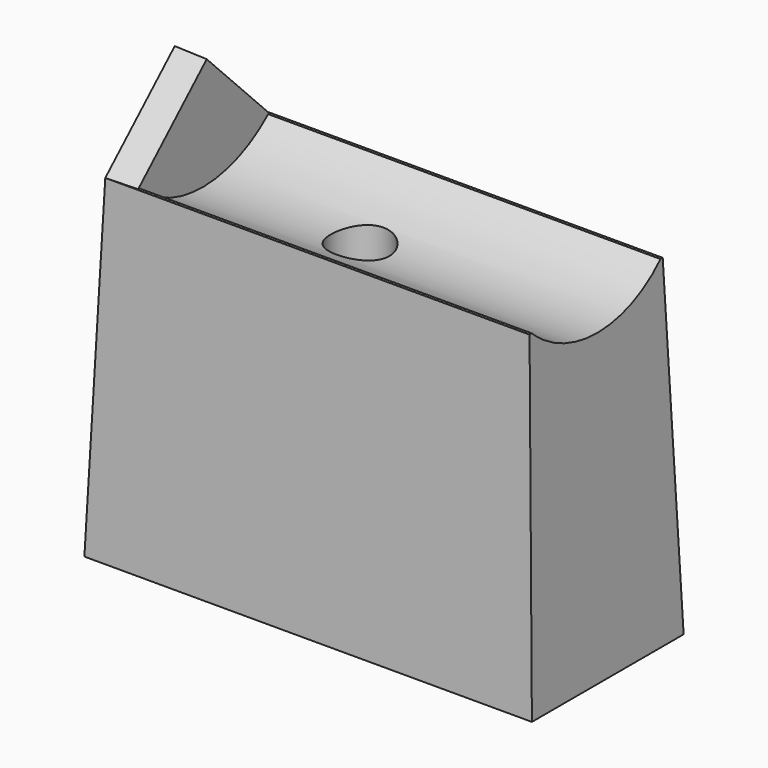
from build123d import *

# Parameters (mm, degrees)
F0_W     = 42
F0_H     = 17.8
F1_DEPTH = 31.2
F1_TAPER = 2
F2_R     = 11
F3_DEPTH = 25
F5_DEPTH = 3
F6_R     = 2.75
F7_DEPTH = 39.0067140634
F8_R     = 5
F8_R_2   = 2.75
F9_DEPTH = 25
F10_SIZE = 2.24999


# Not quite as in the source:
# - a fillet or chamfer is up to 0.001 mm smaller than in the source, because OpenCascade refuses the exact size


with BuildPart() as f1:
    # F0 (on Top) → F1 (new body)
    with BuildSketch(Plane.XY):
        Rectangle(F0_W, F0_H)
    extrude(amount=F1_DEPTH, taper=F1_TAPER)

    # F2 (on Right) → F3 (cut, symmetric)
    with BuildSketch(Plane.YZ):
        with Locations((0, 39.2)):
            Circle(F2_R)
    extrude(amount=F3_DEPTH, both=True, mode=Mode.SUBTRACT)

    # F4 (on face) → F5 (join)
    with BuildSketch(Plane(origin=(-20.9744225277, 0, 0.7324429743), x_dir=(0, -1, 0), z_dir=(-0.999390827, 0, 0.0348994967))):
        with BuildLine():
            Line((0, 38.2966003432), (-7.8104719919, 30.4861283514))
            Line((-7.8104719919, 30.4861283514), (-7.5498344353, 30.4861283514))
            add(Edge.make_bspline(
                [(7.5498344353, 30.4861283514), (0, 23.3567853482), (-7.5498344353, 30.4861283514)],
                knots=[2.3851362689, 2.3851362689, 2.3851362689, 3.8980490383, 3.8980490383, 3.8980490383], degree=2, weights=[1, 0.7272727273, 1]))
            Line((7.5498344353, 30.4861283514), (7.8104719919, 30.4861283514))
            Line((7.8104719919, 30.4861283514), (0, 38.2966003432))
        make_face()
    extrude(amount=-F5_DEPTH)

    # F6 (on face) → F7 (cut, through all)
    with BuildSketch(Plane(origin=(0, 0, 0), x_dir=(1, 0, 0), z_dir=(0, 0, -1))):
        with Locations((-2.25, 0)):
            Circle(F6_R)
    extrude(amount=-F7_DEPTH, mode=Mode.SUBTRACT)

    # F8 (on face) → F9 (cut)
    with BuildSketch(Plane(origin=(0, 0, 0), x_dir=(1, 0, 0), z_dir=(0, 0, -1))):
        with Locations((-2.25, 0)):
            Circle(F8_R)
        with Locations((-2.25, 0)):
            Circle(F8_R_2, mode=Mode.SUBTRACT)
    extrude(amount=-F9_DEPTH, mode=Mode.SUBTRACT)

    # F10 (size 2.25 in the source; OpenCascade refuses exactly that, so slightly less here)
    f10_edges = [f1.edges().sort_by_distance(p)[0] for p in [
        (-7.25, 0, 25),
    ]]
    chamfer(f10_edges, length=F10_SIZE)


solid = f1.part
